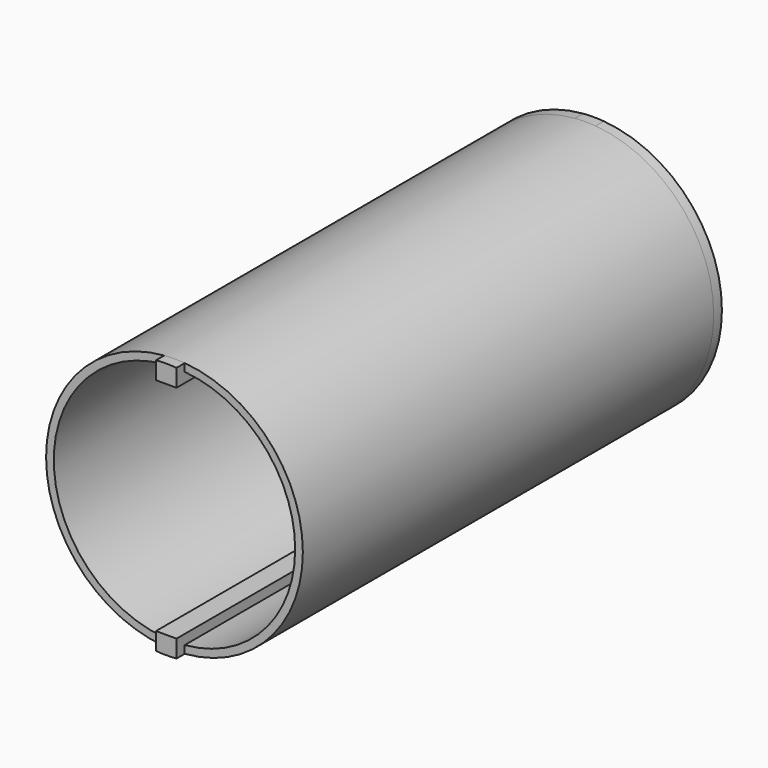
from build123d import *

# Parameters (mm, degrees)
F0_R     = 31.75
F1_DEPTH = 127
F2_R     = 31.75
F2_R_2   = 5.08
F3_DEPTH = 2.54
F5_DEPTH = 2.54
F7_DEPTH = 2.54
F9_DEPTH = 2.54


with BuildPart() as f1:
    # F0 (on Front) → F1 (new body)
    with BuildSketch(Plane.XZ):
        Circle(F0_R)
        with BuildLine():
            ThreePointArc((2.54, 29.7367184639), (21.9832928039, 20.1856102831), (29.845, 0))
            ThreePointArc((29.845, 0), (21.9832928039, -20.1856102831), (2.54, -29.7367184639))
            ThreePointArc((2.54, -29.7367184639), (1.2711535009, -29.817917328), (0, -29.845))
            ThreePointArc((0, -29.845), (-1.2711535009, -29.817917328), (-2.54, -29.7367184639))
            ThreePointArc((-2.54, -29.7367184639), (-29.845, 0), (-2.54, 29.7367184639))
            ThreePointArc((-2.54, 29.7367184639), (-1.2711535009, 29.817917328), (0, 29.845))
            ThreePointArc((0, 29.845), (1.2711535009, 29.817917328), (2.54, 29.7367184639))
        make_face(mode=Mode.SUBTRACT)
        with BuildLine():
            Line((0, 27.305), (0, 29.845))
            ThreePointArc((0, 29.845), (-1.2711535009, 29.817917328), (-2.54, 29.7367184639))
            Line((-2.54, 29.7367184639), (-2.54, 27.305))
            Line((-2.54, 27.305), (0, 27.305))
        make_face()
        with BuildLine():
            Line((2.54, 27.305), (2.54, 29.7367184639))
            ThreePointArc((2.54, 29.7367184639), (1.2711535009, 29.817917328), (0, 29.845))
            Line((0, 29.845), (0, 27.305))
            Line((0, 27.305), (2.54, 27.305))
        make_face()
        with BuildLine():
            ThreePointArc((-2.54, -29.7367184639), (-1.2711535009, -29.817917328), (0, -29.845))
            Line((0, -29.845), (0, -27.305))
            Line((0, -27.305), (-2.54, -27.305))
            Line((-2.54, -27.305), (-2.54, -29.7367184639))
        make_face()
        with BuildLine():
            ThreePointArc((0, -29.845), (1.2711535009, -29.817917328), (2.54, -29.7367184639))
            Line((2.54, -29.7367184639), (2.54, -27.305))
            Line((2.54, -27.305), (0, -27.305))
            Line((0, -27.305), (0, -29.845))
        make_face()
    extrude(amount=F1_DEPTH)

    # F6 (on face) → F7 (join)
    with BuildSketch(Plane(origin=(0, 0, 0), x_dir=(-1, 0, 0), z_dir=(0, 1, 0))):
        with BuildLine():
            Line((-2.54, 29.7367184639), (-2.54, 27.305))
            Line((-2.54, 27.305), (2.54, 27.305))
            Line((2.54, 27.305), (2.54, 29.7367184639))
            Line((2.54, 29.7367184639), (2.54, 31.6482369177))
            ThreePointArc((2.54, 31.6482369177), (0, 31.75), (-2.54, 31.6482369177))
            Line((-2.54, 31.6482369177), (-2.54, 29.7367184639))
        make_face()
        with BuildLine():
            Line((-2.54, -27.305), (-2.54, -29.7367184639))
            Line((-2.54, -29.7367184639), (-2.54, -31.6482369177))
            ThreePointArc((-2.54, -31.6482369177), (0, -31.75), (2.54, -31.6482369177))
            Line((2.54, -31.6482369177), (2.54, -29.7367184639))
            Line((2.54, -29.7367184639), (2.54, -27.305))
            Line((2.54, -27.305), (-2.54, -27.305))
        make_face()
    extrude(amount=F7_DEPTH)

    # F8 (on face) → F9 (join)
    with BuildSketch(Plane.XZ.offset(127)):
        with BuildLine():
            Line((2.54, 29.7367184639), (2.54, 31.6482369177))
            ThreePointArc((2.54, 31.6482369177), (0, 31.75), (-2.54, 31.6482369177))
            Line((-2.54, 31.6482369177), (-2.54, 29.7367184639))
            Line((-2.54, 29.7367184639), (-2.54, 27.305))
            Line((-2.54, 27.305), (2.54, 27.305))
            Line((2.54, 27.305), (2.54, 29.7367184639))
        make_face()
        with BuildLine():
            ThreePointArc((-2.54, -31.6482369177), (0, -31.75), (2.54, -31.6482369177))
            Line((2.54, -31.6482369177), (2.54, -29.7367184639))
            Line((2.54, -29.7367184639), (2.54, -27.305))
            Line((2.54, -27.305), (-2.54, -27.305))
            Line((-2.54, -27.305), (-2.54, -29.7367184639))
            Line((-2.54, -29.7367184639), (-2.54, -31.6482369177))
        make_face()
    extrude(amount=F9_DEPTH)


with BuildPart() as f3:
    # F2 (on Front) → F3 (new body)
    with BuildSketch(Plane.XZ):
        Circle(F2_R)
        Circle(F2_R_2, mode=Mode.SUBTRACT)
    extrude(amount=-F3_DEPTH)

    # F4 (on face) → F5 (cut)
    with BuildSketch(Plane(origin=(0, 2.54, 0), x_dir=(-1, 0, 0), z_dir=(0, 1, 0))):
        with BuildLine():
            ThreePointArc((-2.54, -31.6482369177), (0, -31.75), (2.54, -31.6482369177))
            Line((2.54, -31.6482369177), (2.54, -27.305))
            Line((2.54, -27.305), (0, -27.305))
            Line((0, -27.305), (-2.54, -27.305))
            Line((-2.54, -27.305), (-2.54, -31.6482369177))
        make_face()
        with BuildLine():
            Line((0, 27.305), (0, 31.75))
            ThreePointArc((0, 31.75), (-1.2710188556, 31.7245490286), (-2.54, 31.6482369177))
            Line((-2.54, 31.6482369177), (-2.54, 27.305))
            Line((-2.54, 27.305), (0, 27.305))
        make_face()
        with BuildLine():
            Line((2.54, 27.305), (2.54, 31.6482369177))
            ThreePointArc((2.54, 31.6482369177), (1.2710188556, 31.7245490286), (0, 31.75))
            Line((0, 31.75), (0, 27.305))
            Line((0, 27.305), (2.54, 27.305))
        make_face()
    extrude(amount=-F5_DEPTH, mode=Mode.SUBTRACT)


solid = Compound([f1.part, f3.part])
